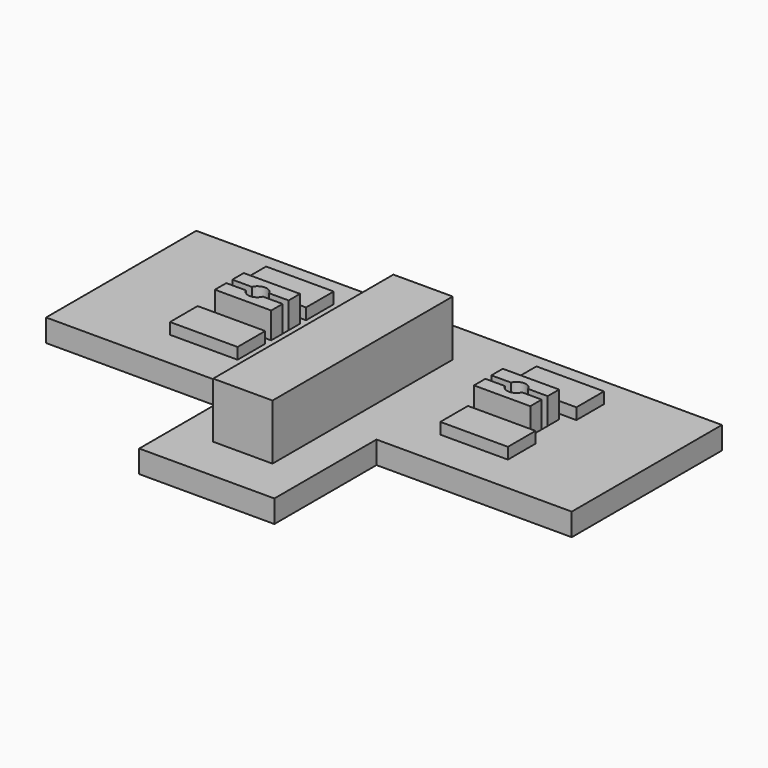
from build123d import *

# Parameters (mm, degrees)
F1_DEPTH = 21
F2_W     = 26
F2_H     = 17
F3_DEPTH = 25
F4_W     = 6
F4_H     = 7.4
F5_DEPTH = 25
F6_W     = 9
F6_H     = 4.6
F7_DEPTH = 1.5
F8_DEPTH = 3.5
F9_DEPTH = 3.001


with BuildPart() as f1:
    # F0 (on Front) → F1 (new body, symmetric)
    with BuildSketch(Plane.XZ):
        Polygon((-35, 0), (35, 0), (35, 3), (3.95, 3), (3.95, 10.4), (0, 10.4), (-3.95, 10.4), (-3.95, 3), (-35, 3), align=None)
    extrude(amount=F1_DEPTH, both=True)

    # F2 (on face) → F3 (cut)
    with BuildSketch(Plane(origin=(0, 0, 0), x_dir=(1, 0, 0), z_dir=(0, 0, -1))):
        with Locations((-22, 12.5)):
            Rectangle(F2_W, F2_H)
        with Locations((22, 12.5)):
            Rectangle(F2_W, F2_H)
    extrude(amount=-F3_DEPTH, mode=Mode.SUBTRACT)

    # F4 (on face) → F5 (cut)
    with BuildSketch(Plane(origin=(-3.95, 0, 0), x_dir=(0, -1, 0), z_dir=(-1, 0, 0))):
        with Locations((-18, 6.7)):
            Rectangle(F4_W, F4_H)
        with Locations((18, 6.7)):
            Rectangle(F4_W, F4_H)
    extrude(amount=-F5_DEPTH, mode=Mode.SUBTRACT)

    # F6 (on face) → F7 (join)
    with BuildSketch(Plane.XY.offset(3)):
        with Locations((-18, 14.7)):
            Rectangle(F6_W, F6_H)
        with Locations((-18, 3.3)):
            Rectangle(F6_W, F6_H)
        with Locations((18, 14.7)):
            Rectangle(F6_W, F6_H)
        with Locations((18, 3.3)):
            Rectangle(F6_W, F6_H)
    extrude(amount=F7_DEPTH)

    # F6 (on face) → F8 (join)
    with BuildSketch(Plane.XY.offset(3)):
        with BuildLine():
            Line((-13.5, 9.5), (-13.5, 11.4))
            Line((-13.5, 11.4), (-21, 11.4))
            Line((-21, 11.4), (-21, 9.5))
            Line((-21, 9.5), (-18.3956439237, 9.5))
            ThreePointArc((-18.3956439237, 9.5), (-17.25, 10.25), (-16.1043560763, 9.5))
            Line((-16.1043560763, 9.5), (-13.5, 9.5))
        make_face()
        with BuildLine():
            Line((-13.5, 6.6), (-13.5, 8.5))
            Line((-13.5, 8.5), (-16.1043560763, 8.5))
            ThreePointArc((-16.1043560763, 8.5), (-17.25, 7.75), (-18.3956439237, 8.5))
            Line((-18.3956439237, 8.5), (-21, 8.5))
            Line((-21, 8.5), (-21, 6.6))
            Line((-21, 6.6), (-13.5, 6.6))
        make_face()
        with BuildLine():
            Line((21, 11.4), (13.5, 11.4))
            Line((13.5, 11.4), (13.5, 9.5))
            Line((13.5, 9.5), (16.1043560763, 9.5))
            ThreePointArc((16.1043560763, 9.5), (17.25, 10.25), (18.3956439237, 9.5))
            Line((18.3956439237, 9.5), (21, 9.5))
            Line((21, 9.5), (21, 11.4))
        make_face()
        with BuildLine():
            Line((13.5, 8.5), (13.5, 6.6))
            Line((13.5, 6.6), (21, 6.6))
            Line((21, 6.6), (21, 8.5))
            Line((21, 8.5), (18.3956439237, 8.5))
            ThreePointArc((18.3956439237, 8.5), (17.25, 7.75), (16.1043560763, 8.5))
            Line((16.1043560763, 8.5), (13.5, 8.5))
        make_face()
    extrude(amount=F8_DEPTH)

    # F6 (on face) → F9 (cut, through all)
    with BuildSketch(Plane.XY.offset(3)):
        with BuildLine():
            Line((-13.5, 8.5), (-13.5, 9.5))
            Line((-13.5, 9.5), (-16.1043560763, 9.5))
            ThreePointArc((-16.1043560763, 9.5), (-16.0263671088, 9.2553870546), (-16, 9))
            ThreePointArc((-16, 9), (-16.0263671088, 8.7446129454), (-16.1043560763, 8.5))
            Line((-16.1043560763, 8.5), (-13.5, 8.5))
        make_face()
        with BuildLine():
            ThreePointArc((-16, 9), (-16.0263671088, 9.2553870546), (-16.1043560763, 9.5))
            Line((-16.1043560763, 9.5), (-18.3956439237, 9.5))
            ThreePointArc((-18.3956439237, 9.5), (-18.5, 9), (-18.3956439237, 8.5))
            Line((-18.3956439237, 8.5), (-16.1043560763, 8.5))
            ThreePointArc((-16.1043560763, 8.5), (-16.0263671088, 8.7446129454), (-16, 9))
        make_face()
        with BuildLine():
            Line((-18.3956439237, 9.5), (-21, 9.5))
            Line((-21, 9.5), (-21, 8.5))
            Line((-21, 8.5), (-18.3956439237, 8.5))
            ThreePointArc((-18.3956439237, 8.5), (-18.5, 9), (-18.3956439237, 9.5))
        make_face()
        with BuildLine():
            Line((16.1043560763, 9.5), (13.5, 9.5))
            Line((13.5, 9.5), (13.5, 8.5))
            Line((13.5, 8.5), (16.1043560763, 8.5))
            ThreePointArc((16.1043560763, 8.5), (16, 9), (16.1043560763, 9.5))
        make_face()
        with BuildLine():
            Line((18.3956439237, 9.5), (16.1043560763, 9.5))
            ThreePointArc((16.1043560763, 9.5), (16, 9), (16.1043560763, 8.5))
            Line((16.1043560763, 8.5), (18.3956439237, 8.5))
            ThreePointArc((18.3956439237, 8.5), (18.4736328912, 8.7446129454), (18.5, 9))
            ThreePointArc((18.5, 9), (18.4736328912, 9.2553870546), (18.3956439237, 9.5))
        make_face()
        with BuildLine():
            Line((21, 8.5), (21, 9.5))
            Line((21, 9.5), (18.3956439237, 9.5))
            ThreePointArc((18.3956439237, 9.5), (18.4736328912, 9.2553870546), (18.5, 9))
            ThreePointArc((18.5, 9), (18.4736328912, 8.7446129454), (18.3956439237, 8.5))
            Line((18.3956439237, 8.5), (21, 8.5))
        make_face()
        with BuildLine():
            Line((-18.3956439237, 9.5), (-16.1043560763, 9.5))
            ThreePointArc((-16.1043560763, 9.5), (-17.25, 10.25), (-18.3956439237, 9.5))
        make_face()
        with BuildLine():
            ThreePointArc((-18.3956439237, 8.5), (-17.25, 7.75), (-16.1043560763, 8.5))
            Line((-16.1043560763, 8.5), (-18.3956439237, 8.5))
        make_face()
        with BuildLine():
            ThreePointArc((18.3956439237, 9.5), (17.25, 10.25), (16.1043560763, 9.5))
            Line((16.1043560763, 9.5), (18.3956439237, 9.5))
        make_face()
        with BuildLine():
            Line((18.3956439237, 8.5), (16.1043560763, 8.5))
            ThreePointArc((16.1043560763, 8.5), (17.25, 7.75), (18.3956439237, 8.5))
        make_face()
    extrude(amount=-F9_DEPTH, mode=Mode.SUBTRACT)


solid = f1.part
